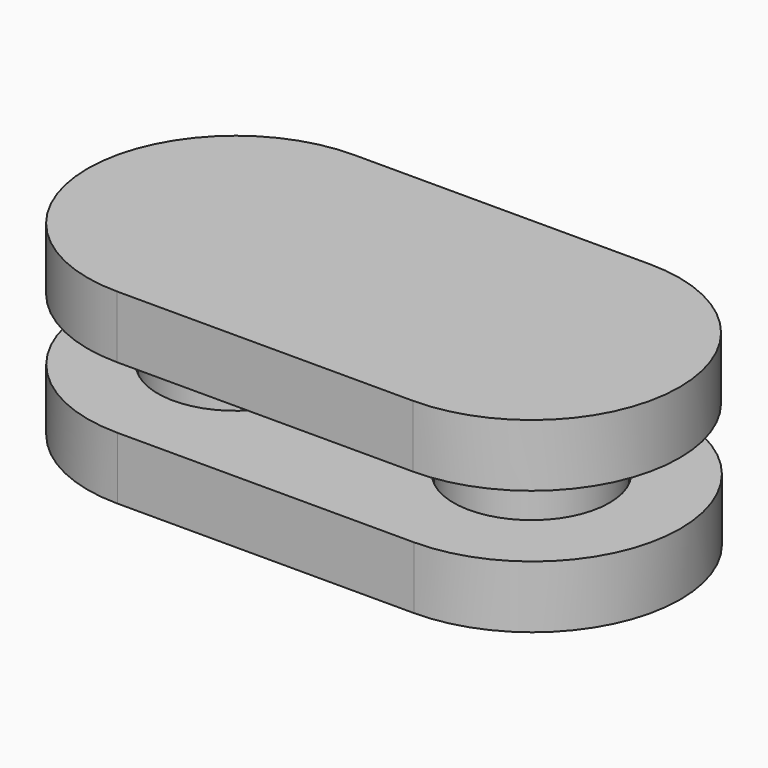
from build123d import *

# Parameters (mm, degrees)
F0_R          = 1.25
F0_R_2        = 1.225
F1_DEPTH      = 1
F2_DEPTH      = 1.5
F3_R          = 1.225
F4_DEPTH      = 0.5
F4_DEPTH_BACK = 0.5
F5_DEPTH      = 1.5
F6_DEPTH      = 1.45


with BuildPart() as f1:
    # F0 (on Top) → F1 (new body)
    with BuildSketch(Plane.XY):
        with BuildLine():
            Line((0.2638664927, -2.3833251961), (2.6388664927, -2.3833251961))
            ThreePointArc((2.6388664927, -2.3833251961), (5.0138664949, -0.0082244105), (2.6386649301, 2.3666748038))
            Line((2.6386649301, 2.3666748038), (0.2638664927, 2.3664732583))
            Line((0.2638664927, 2.3664732497), (-2.1109319446, 2.3666747953))
            ThreePointArc((-2.1109319446, 2.3666747953), (-4.4861335051, -0.0082244148), (-2.1111335073, -2.3833251962))
            Line((-2.1111335073, -2.3833251962), (0.2638664927, -2.3833251962))
        make_face()
        with Locations((-2.1111335073, -0.0083251962)):
            Circle(F0_R, mode=Mode.SUBTRACT)
        with Locations((2.6388664927, -0.0083251919)):
            Circle(F0_R, mode=Mode.SUBTRACT)
        with Locations((2.6388664927, -0.0083251919)):
            Circle(F0_R)
        with Locations((2.6388664927, -0.0083251919)):
            Circle(F0_R_2, mode=Mode.SUBTRACT)
        with Locations((-2.1111335073, -0.0083251962)):
            Circle(F0_R)
        with Locations((-2.1111335073, -0.0083251962)):
            Circle(F0_R_2, mode=Mode.SUBTRACT)
        with Locations((-2.1111335073, -0.0083251962)):
            Circle(F0_R_2)
        with Locations((2.6388664927, -0.0083251919)):
            Circle(F0_R_2)
    extrude(amount=F1_DEPTH)

    # F0 (on Top) → F2 (join)
    with BuildSketch(Plane.XY):
        with Locations((2.6388664927, -0.0083251919)):
            Circle(F0_R_2)
        with Locations((-2.1111335073, -0.0083251962)):
            Circle(F0_R_2)
    extrude(amount=-F2_DEPTH)


with BuildPart() as f4:
    # F3 (on face) → F4 (new body, two sides)
    with BuildSketch(Plane(origin=(0, 0, -1.5), x_dir=(1, 0, 0), z_dir=(0, 0, -1))) as f4_sk:
        with BuildLine():
            Line((2.6456569321, 2.375), (-2.1152956275, 2.375))
            ThreePointArc((-2.1152956275, 2.375), (-4.4902956275, 0), (-2.1152956275, -2.375))
            Line((-2.1152956275, -2.375), (2.6456569321, -2.375))
            ThreePointArc((2.6456569321, -2.375), (5.0206569321, 0), (2.6456569321, 2.375))
        make_face()
        with Locations((-2.1111335073, 0.0083251962)):
            Circle(F3_R, mode=Mode.SUBTRACT)
        with Locations((-2.1111335073, 0.0083251962)):
            Circle(F3_R)
    extrude(amount=F4_DEPTH)
    extrude(f4_sk.sketch, amount=-F4_DEPTH_BACK)


with BuildPart() as f5_tool:
    # F0 (on Top) → F5 (new body)
    with BuildSketch(Plane.XY):
        with Locations((2.6388664927, -0.0083251919)):
            Circle(F0_R)
        with Locations((2.6388664927, -0.0083251919)):
            Circle(F0_R_2, mode=Mode.SUBTRACT)
        with Locations((-2.1111335073, -0.0083251962)):
            Circle(F0_R)
        with Locations((-2.1111335073, -0.0083251962)):
            Circle(F0_R_2, mode=Mode.SUBTRACT)
        with Locations((2.6388664927, -0.0083251919)):
            Circle(F0_R_2)
        with Locations((-2.1111335073, -0.0083251962)):
            Circle(F0_R_2)
    extrude(amount=-F5_DEPTH)


with BuildPart() as f1_1:
    add(f1.part)

    # F5: cut by f5_tool
    add(f5_tool.part, mode=Mode.SUBTRACT)

    # F0 (on Top) → F6 (join)
    with BuildSketch(Plane.XY):
        with Locations((2.6388664927, -0.0083251919)):
            Circle(F0_R_2)
        with Locations((-2.1111335073, -0.0083251962)):
            Circle(F0_R_2)
    extrude(amount=-F6_DEPTH)


with BuildPart() as f4_1:
    add(f4.part)

    # F5: cut by f5_tool
    add(f5_tool.part, mode=Mode.SUBTRACT)


solid = Compound([f1_1.part, f4_1.part])
